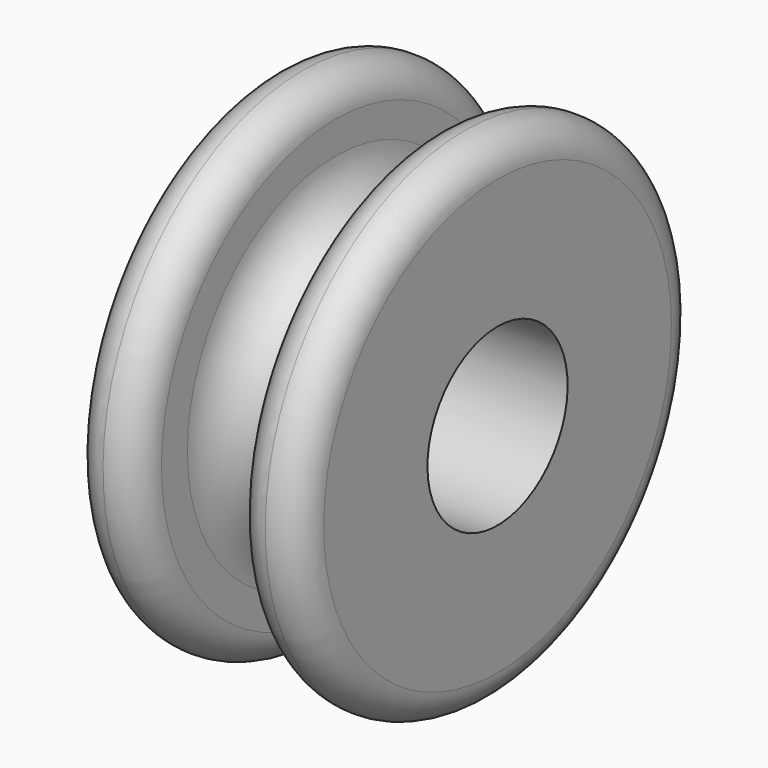
from build123d import *

# Parameters (mm, degrees)
F2_R = 0.99999


# Not quite as in the source:
# - a fillet or chamfer is up to 0.001 mm smaller than in the source, because OpenCascade refuses the exact size


with BuildPart() as f1:
    # F0 (on Front) → F1 (revolve)
    with BuildSketch(Plane.XZ):
        with BuildLine():
            Line((0, 7.7), (0, 2.7))
            Line((0, 2.7), (7, 2.7))
            Line((7, 2.7), (7, 7.7))
            Line((7, 7.7), (5, 7.7))
            Line((5, 7.7), (5, 5.7))
            ThreePointArc((5, 5.7), (3.5, 4.2), (2, 5.7))
            Line((2, 5.7), (2, 7.7))
            Line((2, 7.7), (0, 7.7))
        make_face()
    revolve(axis=Axis((3.5, 0, 0), (1, 0, 0)))

    # F2 (radius 1 in the source; OpenCascade refuses exactly that, so slightly less here)
    f2_edges = [f1.edges().sort_by_distance(p)[0] for p in [
        (7, 0, -7.7),
        (5, 0, -7.7),
        (2, 0, -7.7),
        (0, 0, -7.7),
    ]]
    fillet(f2_edges, radius=F2_R)


solid = f1.part
